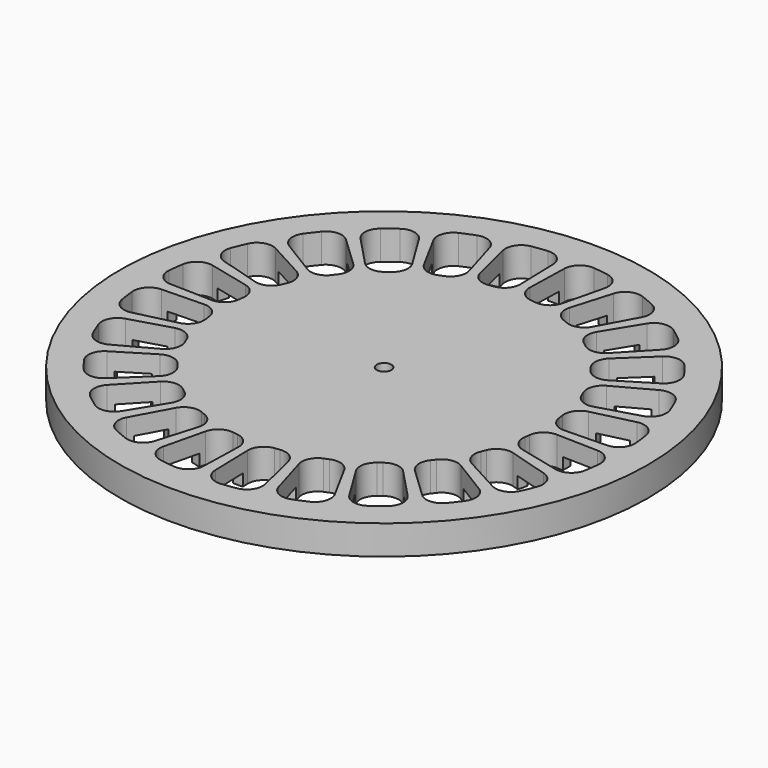
from build123d import *

# Parameters (mm, degrees)
F0_R            = 114.3
F1_DEPTH        = 12.7
F2_R            = 63.5
F3_DEPTH        = 7.62
F5_DEPTH        = 12.701
F5_COPIES_COUNT = 24
F6_R            = 3.175
F7_DEPTH        = 12.701
F8_R            = 91.7971404603
F8_R_2          = 79.0971404603
F9_DEPTH        = 5.08


# Not quite as in the source:
# - a pattern or mirror of a feature is missing from the dataset's text; its kind, count and spacing are read off the source's solid


with BuildPart() as f1:
    # F0 (on Top) → F1 (new body)
    with BuildSketch(Plane.XY):
        Circle(F0_R)
    extrude(amount=F1_DEPTH)

    # F2 (on Top) → F3 (cut, through all)
    with BuildSketch(Plane.XY):
        Circle(F2_R)
    extrude(amount=F3_DEPTH, mode=Mode.SUBTRACT)

    # F4 (on face) → F5 (cut, through all)
    with BuildSketch(Plane(origin=(0, 0, 0), x_dir=(1, 0, 0), z_dir=(0, 0, -1))):
        with BuildLine():
            ThreePointArc((2.4735504756, -94.4610816582), (4.7917264077, -99.423883909), (10.0045044615, -101.1062307204))
            ThreePointArc((10.0045044615, -101.1062307204), (13.2614611296, -100.7307979156), (16.5046088504, -100.250475743))
            ThreePointArc((16.5046088504, -100.250475743), (21.104342404, -97.2762872709), (22.0590606671, -91.882600325))
            Line((22.0590606671, -91.882600325), (17.8354169233, -74.2898580102))
            ThreePointArc((17.8354169233, -74.2898580102), (15.0082627527, -70.209618081), (10.168538419, -69.1058848899))
            ThreePointArc((10.168538419, -69.1058848899), (9.1172545266, -69.252423567), (8.0638652637, -69.3829703674))
            ThreePointArc((8.0638652637, -69.3829703674), (3.6747177081, -71.7017075927), (1.9999402821, -76.3746380605))
            Line((1.9999402821, -76.3746380605), (2.4735504756, -94.4610816582))
        make_face()
    f5 = extrude(amount=-F5_DEPTH, mode=Mode.SUBTRACT)

    # F5_copies: F5 ×24 about axis
    f5_copies_axis = Axis((0, 0, 0), (0, 0, 1))
    for i in range(1, F5_COPIES_COUNT):
        add(f5.rotate(f5_copies_axis, i * 360 / F5_COPIES_COUNT), mode=Mode.SUBTRACT)

    # F6 (on face) → F7 (cut, through all)
    with BuildSketch(Plane.XY.offset(12.7)):
        Circle(F6_R)
    extrude(amount=-F7_DEPTH, mode=Mode.SUBTRACT)

    # F8 (on face) → F9 (cut)
    with BuildSketch(Plane(origin=(0, 0, 0), x_dir=(1, 0, 0), z_dir=(0, 0, -1))):
        Circle(F8_R)
        Circle(F8_R_2, mode=Mode.SUBTRACT)
    extrude(amount=-F9_DEPTH, mode=Mode.SUBTRACT)


solid = f1.part
